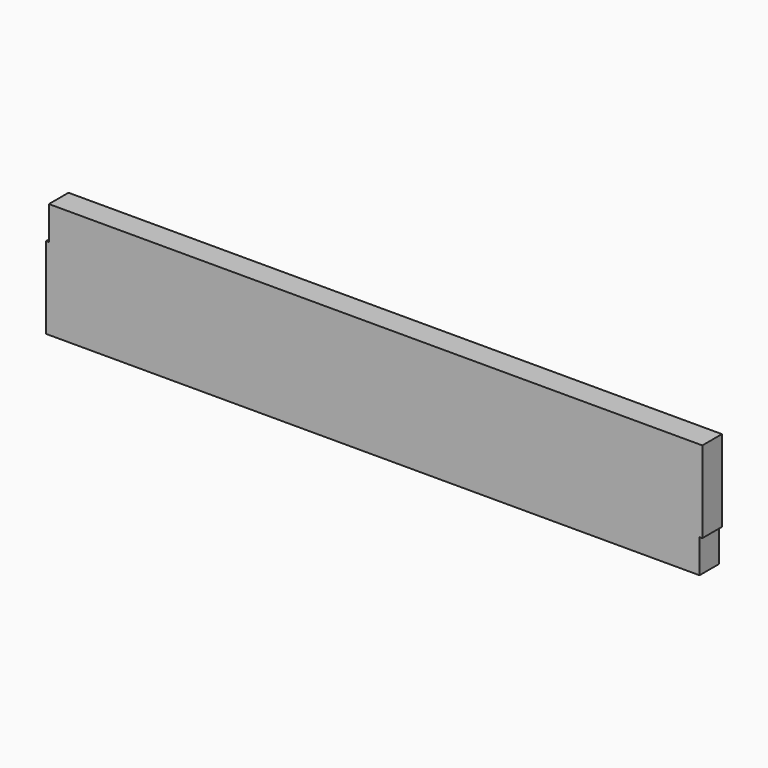
from build123d import *

# Parameters (mm, degrees)
F0_W     = 505.8128448129
F0_H     = 37.4025163994
F1_DEPTH = 9.525


# Not quite as in the source:
# - the program builds the solid bodies; features that only make, move or delete a surface that nothing else refers to are left out


with BuildPart() as f1:
    # F0 (on Front) → F1 (new body, symmetric)
    with BuildSketch(Plane.XZ):
        Polygon((-254, 5.6525163994), (-256.1871551871, 5.6525163994), (-256.1871551871, -57.8474836006), (251.8128448129, -57.8474836006), (251.8128448129, -31.75), (-254, -31.75), align=None)
        Polygon((-254, 31.75), (-254, 5.6525163994), (251.8128448129, 5.6525163994), (251.8128448129, -31.75), (254, -31.75), (254, 31.75), align=None)
        with Locations((-1.0935775936, -13.0487418003)):
            Rectangle(F0_W, F0_H)
    extrude(amount=F1_DEPTH, both=True)


solid = f1.part
